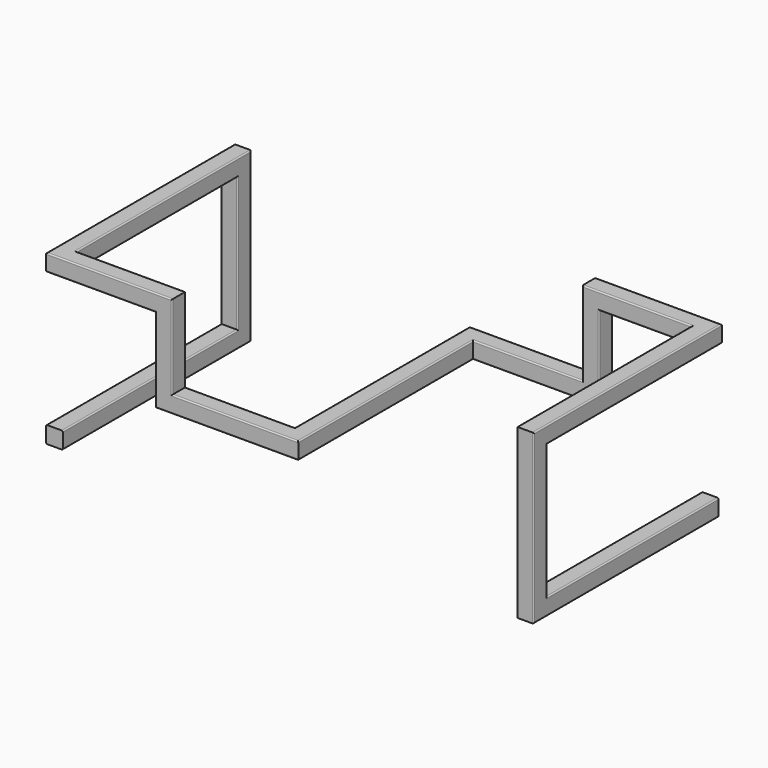
from build123d import *

# Parameters (mm, degrees)
F0_W      = 40
F0_H      = 40
F1_DEPTH  = 560
F2_W      = 40
F2_H      = 40
F3_DEPTH  = 360
F4_W      = 40
F4_H      = 40
F5_DEPTH  = 520
F6_W      = 40
F6_H      = 40
F7_DEPTH  = 260
F8_W      = 40
F8_H      = 40
F9_DEPTH  = 200
F10_W     = 40
F10_H     = 40
F11_DEPTH = 300
F12_W     = 40
F12_H     = 40
F13_DEPTH = 520
F14_W     = 40
F14_H     = 40
F15_DEPTH = 300
F16_W     = 40
F16_H     = 40
F17_DEPTH = 200
F18_W     = 40
F18_H     = 40
F19_DEPTH = 260
F20_W     = 40
F20_H     = 40
F21_DEPTH = 520
F22_W     = 40
F22_H     = 40
F23_DEPTH = 360
F24_W     = 40
F24_H     = 40
F25_DEPTH = 510
F26_R     = 3


with BuildPart() as f1:
    # F0 (on Front) → F1 (new body)
    with BuildSketch(Plane.XZ):
        with Locations((20, 20)):
            Rectangle(F0_W, F0_H)
    extrude(amount=-F1_DEPTH)

    # F2 (on face) → F3 (join)
    with BuildSketch(Plane.XY.offset(40)):
        with Locations((20, 540)):
            Rectangle(F2_W, F2_H)
    extrude(amount=F3_DEPTH)

    # F4 (on face) → F5 (join)
    with BuildSketch(Plane.XZ.offset(-520)):
        with Locations((20, 380)):
            Rectangle(F4_W, F4_H)
    extrude(amount=F5_DEPTH)

    # F6 (on face) → F7 (join)
    with BuildSketch(Plane.YZ.offset(40)):
        with Locations((20, 380)):
            Rectangle(F6_W, F6_H)
    extrude(amount=F7_DEPTH)

    # F8 (on face) → F9 (join)
    with BuildSketch(Plane(origin=(0, 0, 360), x_dir=(1, 0, 0), z_dir=(0, 0, -1))):
        with Locations((280, -20)):
            Rectangle(F8_W, F8_H)
    extrude(amount=F9_DEPTH)

    # F10 (on face) → F11 (join)
    with BuildSketch(Plane.YZ.offset(300)):
        with Locations((20, 180)):
            Rectangle(F10_W, F10_H)
    extrude(amount=F11_DEPTH)

    # F12 (on face) → F13 (join)
    with BuildSketch(Plane(origin=(0, 40, 0), x_dir=(-1, 0, 0), z_dir=(0, 1, 0))):
        with Locations((-580, 180)):
            Rectangle(F12_W, F12_H)
    extrude(amount=F13_DEPTH)

    # F14 (on face) → F15 (join)
    with BuildSketch(Plane.YZ.offset(600)):
        with Locations((540, 180)):
            Rectangle(F14_W, F14_H)
    extrude(amount=F15_DEPTH)

    # F16 (on face) → F17 (join)
    with BuildSketch(Plane.XY.offset(200)):
        with Locations((880, 540)):
            Rectangle(F16_W, F16_H)
    extrude(amount=F17_DEPTH)

    # F18 (on face) → F19 (join)
    with BuildSketch(Plane.YZ.offset(900)):
        with Locations((540, 380)):
            Rectangle(F18_W, F18_H)
    extrude(amount=F19_DEPTH)

    # F20 (on face) → F21 (join)
    with BuildSketch(Plane.XZ.offset(-520)):
        with Locations((1140, 380)):
            Rectangle(F20_W, F20_H)
    extrude(amount=F21_DEPTH)

    # F22 (on face) → F23 (join)
    with BuildSketch(Plane(origin=(0, 0, 360), x_dir=(1, 0, 0), z_dir=(0, 0, -1))):
        with Locations((1140, -20)):
            Rectangle(F22_W, F22_H)
    extrude(amount=F23_DEPTH)

    # F24 (on face) → F25 (join)
    with BuildSketch(Plane(origin=(0, 40, 0), x_dir=(-1, 0, 0), z_dir=(0, 1, 0))):
        with Locations((-1140, 20)):
            Rectangle(F24_W, F24_H)
    extrude(amount=F25_DEPTH)

    # F26
    f26_edges = [f1.edges().sort_by_distance(p)[0] for p in [
        (0, 280, 400),
        (150, 0, 400),
        (170, 40, 400),
        (40, 300, 400),
        (0, 260, 40),
        (130, 0, 360),
        (260, 0, 260),
        (300, 0, 300),
        (430, 40, 200),
        (450, 0, 200),
        (430, 0, 160),
        (40, 520, 200),
        (0, 560, 200),
        (0, 280, 0),
        (40, 260, 40),
        (560, 300, 200),
        (600, 260, 200),
        (710, 560, 200),
        (730, 520, 200),
        (750, 520, 160),
        (560, 300, 160),
        (1120, 275, 0),
        (1160, 295, 40),
        (1120, 295, 40),
        (1120, 40, 200),
        (1160, 0, 200),
        (1120, 0, 200),
        (1120, 280, 360),
        (1160, 280, 400),
        (1120, 260, 400),
        (1010, 560, 400),
        (990, 520, 400),
        (1010, 520, 360),
        (900, 520, 260),
        (860, 520, 300),
        (860, 560, 300),
        (1160, 300, 360),
        (1160, 275, 0),
        (1030, 560, 360),
        (730, 560, 160),
        (900, 560, 260),
        (600, 260, 160),
        (410, 40, 160),
        (150, 40, 360),
        (300, 40, 300),
        (1160, 40, 200),
        (40, 560, 200),
        (40, 280, 0),
        (0, 520, 200),
        (0, 260, 360),
        (40, 280, 360),
        (260, 40, 260),
    ]]
    fillet(f26_edges, radius=F26_R)


solid = f1.part
